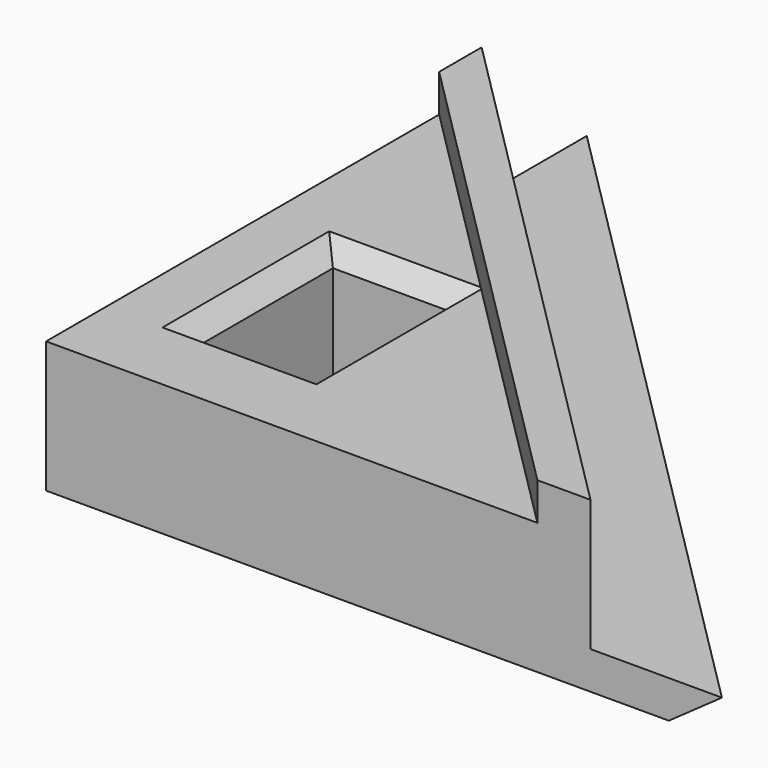
from build123d import *

# Parameters (mm, degrees)
F1_DEPTH     = 2
F3_DEPTH     = 5
F5_DEPTH     = 2
F6_W         = 6.2
F6_H         = 9.1
F7_DEPTH     = 7.001
F8_T1_DEPTH  = 9.1
F8_T3_DEPTH  = 6.2
F8_T9_DEPTH  = 8.771682988
F8_T13_DEPTH = 11.671682988
F8_T20_DEPTH = 11.671682988
F8_T24_DEPTH = 8.771682988
F8_T31_DEPTH = 8.771682988
F8_T36_DEPTH = 11.671682988
F8_T44_DEPTH = 8.771682988
F8_T48_DEPTH = 11.671682988
F8_T55_DEPTH = 8.771682988
F8_T59_DEPTH = 11.671682988
F8_T66_DEPTH = 8.771682988
F8_T70_DEPTH = 11.671682988
F8_T77_DEPTH = 8.771682988
F8_T81_DEPTH = 11.671682988
F8_T88_DEPTH = 11.671682988
F8_T92_DEPTH = 8.771682988
F9_SIZE      = 1.99999


# Not quite as in the source:
# - a fillet or chamfer that OpenCascade refuses, or shapes differently, is made with other operations: its cross-section is extruded or revolved along the edge and cut away or added
# - a fillet or chamfer is up to 0.001 mm smaller than in the source, because OpenCascade refuses the exact size


with BuildPart() as f1:
    # F0 (on Top) → F1 (new body)
    with BuildSketch(Plane.XY):
        Polygon((0, 36), (0, 0), (36, 0), align=None)
    extrude(amount=F1_DEPTH)

    # F2 (on face) → F3 (join)
    with BuildSketch(Plane.XY.offset(2)):
        Polygon((0, 29), (0, 0), (29, 0), align=None)
    extrude(amount=F3_DEPTH)

    # F4 (on face) → F5 (join)
    with BuildSketch(Plane.XY.offset(7)):
        Polygon((29, 0), (0, 29), (0, 26.1715728753), (26.1715728753, 0), align=None)
    extrude(amount=F5_DEPTH)

    # F6 (on face) → F7 (cut, through all)
    with BuildSketch(Plane.XY.offset(7)):
        with Locations((7.1, 9.55)):
            Rectangle(F6_W, F6_H)
    extrude(amount=-F7_DEPTH, mode=Mode.SUBTRACT)

    # F8: chamfer of 1 on 8 edges, made by hand

    # F8_s2 → F8_t1 (cut)
    with BuildSketch(Plane.XZ.offset(-14.1)):
        Polygon((3, 7), (4, 6), (4, 7), align=None)
        Polygon((11.2, 7), (10.2, 6), (10.2, 7), align=None)
        Polygon((11.2, 0), (10.2, 1), (10.2, 0), align=None)
        Polygon((3, 0), (4, 1), (4, 0), align=None)
    extrude(amount=F8_T1_DEPTH, mode=Mode.SUBTRACT)

    # F8_s4 → F8_t3 (cut)
    with BuildSketch(Plane.YZ.offset(4)):
        Polygon((15.1, 7), (14.1, 6), (14.1, 7), align=None)
        Polygon((4, 7), (5, 6), (5, 7), align=None)
        Polygon((15.1, 0), (14.1, 1), (14.1, 0), align=None)
        Polygon((4, 0), (5, 1), (5, 0), align=None)
    extrude(amount=F8_T3_DEPTH, mode=Mode.SUBTRACT)


with BuildPart() as f8_tool7:
    # F8_s8 → F8_t9 (new body)
    with BuildSketch(Plane.YZ.offset(10.2)):
        Polygon((15.1, 7), (14.1, 6), (14.1, 7), align=None)
    extrude(amount=-F8_T9_DEPTH)

    split(bisect_by=Plane.YZ.offset(4), keep=Keep.BOTTOM)


with BuildPart() as f8_tool11:
    # F8_s12 → F8_t13 (new body)
    with BuildSketch(Plane.XZ.offset(-16.671682988)):
        Polygon((3, 7), (4, 6), (4, 7), align=None)
    extrude(amount=F8_T13_DEPTH)

    split(bisect_by=Plane.XZ.offset(-14.1), keep=Keep.BOTTOM)


with BuildPart() as f8_tool7_1:
    add(f8_tool7.part)

    # F8_t15: intersect F8_tool11
    add(f8_tool11.part, mode=Mode.INTERSECT)


with BuildPart() as f1_1:
    add(f1.part)

    # F8_t5: cut F8_tool7
    add(f8_tool7_1.part, mode=Mode.SUBTRACT)


with BuildPart() as f8_tool18:
    # F8_s19 → F8_t20 (new body)
    with BuildSketch(Plane.XZ.offset(-14.1)):
        Polygon((3, 7), (4, 6), (4, 7), align=None)
    extrude(amount=F8_T20_DEPTH)

    split(bisect_by=Plane.XZ.offset(-5), keep=Keep.TOP)


with BuildPart() as f8_tool22:
    # F8_s23 → F8_t24 (new body)
    with BuildSketch(Plane.YZ.offset(1.428317012)):
        Polygon((4, 7), (5, 6), (5, 7), align=None)
    extrude(amount=F8_T24_DEPTH)

    split(bisect_by=Plane.YZ.offset(4), keep=Keep.BOTTOM)


with BuildPart() as f8_tool18_1:
    add(f8_tool18.part)

    # F8_t26: intersect F8_tool22
    add(f8_tool22.part, mode=Mode.INTERSECT)


with BuildPart() as f1_2:
    add(f1_1.part)

    # F8_t16: cut F8_tool18
    add(f8_tool18_1.part, mode=Mode.SUBTRACT)


with BuildPart() as f8_tool29:
    # F8_s30 → F8_t31 (new body)
    with BuildSketch(Plane.YZ.offset(12.771682988)):
        Polygon((15.1, 7), (14.1, 6), (14.1, 7), align=None)
    extrude(amount=-F8_T31_DEPTH)

    split(bisect_by=Plane(origin=(13.0857864376, 13.0857864376, 0), x_dir=(0, 0, 1), z_dir=(-0.7071067812, -0.7071067812, 0)), keep=Keep.TOP)

    split(bisect_by=Plane.YZ.offset(10.2), keep=Keep.TOP)


with BuildPart() as f8_tool34:
    # F8_s35 → F8_t36 (new body)
    with BuildSketch(Plane.XZ.offset(-5)):
        Polygon((11.2, 7), (10.2, 6), (10.2, 7), align=None)
    extrude(amount=-F8_T36_DEPTH)

    split(bisect_by=Plane(origin=(13.0857864376, 13.0857864376, 0), x_dir=(0, 0, 1), z_dir=(-0.7071067812, -0.7071067812, 0)), keep=Keep.TOP)

    split(bisect_by=Plane.XZ.offset(-14.1), keep=Keep.BOTTOM)


with BuildPart() as f8_tool29_1:
    add(f8_tool29.part)

    # F8_t39: intersect F8_tool34
    add(f8_tool34.part, mode=Mode.INTERSECT)


with BuildPart() as f1_3:
    add(f1_2.part)

    # F8_t27: cut F8_tool29
    add(f8_tool29_1.part, mode=Mode.SUBTRACT)


with BuildPart() as f8_tool42:
    # F8_s43 → F8_t44 (new body)
    with BuildSketch(Plane.YZ.offset(4)):
        Polygon((4, 7), (5, 6), (5, 7), align=None)
    extrude(amount=F8_T44_DEPTH)

    split(bisect_by=Plane.YZ.offset(10.2), keep=Keep.TOP)


with BuildPart() as f8_tool46:
    # F8_s47 → F8_t48 (new body)
    with BuildSketch(Plane.XZ.offset(-2.428317012)):
        Polygon((11.2, 7), (10.2, 6), (10.2, 7), align=None)
    extrude(amount=-F8_T48_DEPTH)

    split(bisect_by=Plane.XZ.offset(-5), keep=Keep.TOP)


with BuildPart() as f8_tool42_1:
    add(f8_tool42.part)

    # F8_t50: intersect F8_tool46
    add(f8_tool46.part, mode=Mode.INTERSECT)


with BuildPart() as f1_4:
    add(f1_3.part)

    # F8_t40: cut F8_tool42
    add(f8_tool42_1.part, mode=Mode.SUBTRACT)


with BuildPart() as f8_tool53:
    # F8_s54 → F8_t55 (new body)
    with BuildSketch(Plane.YZ.offset(12.771682988)):
        Polygon((15.1, 0), (14.1, 1), (14.1, 0), align=None)
    extrude(amount=-F8_T55_DEPTH)

    split(bisect_by=Plane.YZ.offset(10.2), keep=Keep.TOP)


with BuildPart() as f8_tool57:
    # F8_s58 → F8_t59 (new body)
    with BuildSketch(Plane.XZ.offset(-5)):
        Polygon((11.2, 0), (10.2, 1), (10.2, 0), align=None)
    extrude(amount=-F8_T59_DEPTH)

    split(bisect_by=Plane.XZ.offset(-14.1), keep=Keep.BOTTOM)


with BuildPart() as f8_tool53_1:
    add(f8_tool53.part)

    # F8_t61: intersect F8_tool57
    add(f8_tool57.part, mode=Mode.INTERSECT)


with BuildPart() as f1_5:
    add(f1_4.part)

    # F8_t51: cut F8_tool53
    add(f8_tool53_1.part, mode=Mode.SUBTRACT)


with BuildPart() as f8_tool64:
    # F8_s65 → F8_t66 (new body)
    with BuildSketch(Plane.YZ.offset(10.2)):
        Polygon((15.1, 0), (14.1, 1), (14.1, 0), align=None)
    extrude(amount=-F8_T66_DEPTH)

    split(bisect_by=Plane.YZ.offset(4), keep=Keep.BOTTOM)


with BuildPart() as f8_tool68:
    # F8_s69 → F8_t70 (new body)
    with BuildSketch(Plane.XZ.offset(-16.671682988)):
        Polygon((3, 0), (4, 1), (4, 0), align=None)
    extrude(amount=F8_T70_DEPTH)

    split(bisect_by=Plane.XZ.offset(-14.1), keep=Keep.BOTTOM)


with BuildPart() as f8_tool64_1:
    add(f8_tool64.part)

    # F8_t72: intersect F8_tool68
    add(f8_tool68.part, mode=Mode.INTERSECT)


with BuildPart() as f1_6:
    add(f1_5.part)

    # F8_t62: cut F8_tool64
    add(f8_tool64_1.part, mode=Mode.SUBTRACT)


with BuildPart() as f8_tool75:
    # F8_s76 → F8_t77 (new body)
    with BuildSketch(Plane.YZ.offset(4)):
        Polygon((4, 0), (5, 1), (5, 0), align=None)
    extrude(amount=F8_T77_DEPTH)

    split(bisect_by=Plane.YZ.offset(10.2), keep=Keep.TOP)


with BuildPart() as f8_tool79:
    # F8_s80 → F8_t81 (new body)
    with BuildSketch(Plane.XZ.offset(-2.428317012)):
        Polygon((11.2, 0), (10.2, 1), (10.2, 0), align=None)
    extrude(amount=-F8_T81_DEPTH)

    split(bisect_by=Plane.XZ.offset(-5), keep=Keep.TOP)


with BuildPart() as f8_tool75_1:
    add(f8_tool75.part)

    # F8_t83: intersect F8_tool79
    add(f8_tool79.part, mode=Mode.INTERSECT)


with BuildPart() as f1_7:
    add(f1_6.part)

    # F8_t73: cut F8_tool75
    add(f8_tool75_1.part, mode=Mode.SUBTRACT)


with BuildPart() as f8_tool86:
    # F8_s87 → F8_t88 (new body)
    with BuildSketch(Plane.XZ.offset(-14.1)):
        Polygon((3, 0), (4, 1), (4, 0), align=None)
    extrude(amount=F8_T88_DEPTH)

    split(bisect_by=Plane.XZ.offset(-5), keep=Keep.TOP)


with BuildPart() as f8_tool90:
    # F8_s91 → F8_t92 (new body)
    with BuildSketch(Plane.YZ.offset(1.428317012)):
        Polygon((4, 0), (5, 1), (5, 0), align=None)
    extrude(amount=F8_T92_DEPTH)

    split(bisect_by=Plane.YZ.offset(4), keep=Keep.BOTTOM)


with BuildPart() as f8_tool86_1:
    add(f8_tool86.part)

    # F8_t94: intersect F8_tool90
    add(f8_tool90.part, mode=Mode.INTERSECT)


with BuildPart() as f1_8:
    add(f1_7.part)

    # F8_t84: cut F8_tool86
    add(f8_tool86_1.part, mode=Mode.SUBTRACT)

    # F9 (size 2 in the source; OpenCascade refuses exactly that, so slightly less here)
    f9_edges = [f1_8.edges().sort_by_distance(p)[0] for p in [
        (18, 18, 0),
    ]]
    chamfer(f9_edges, length=F9_SIZE)


solid = f1_8.part
